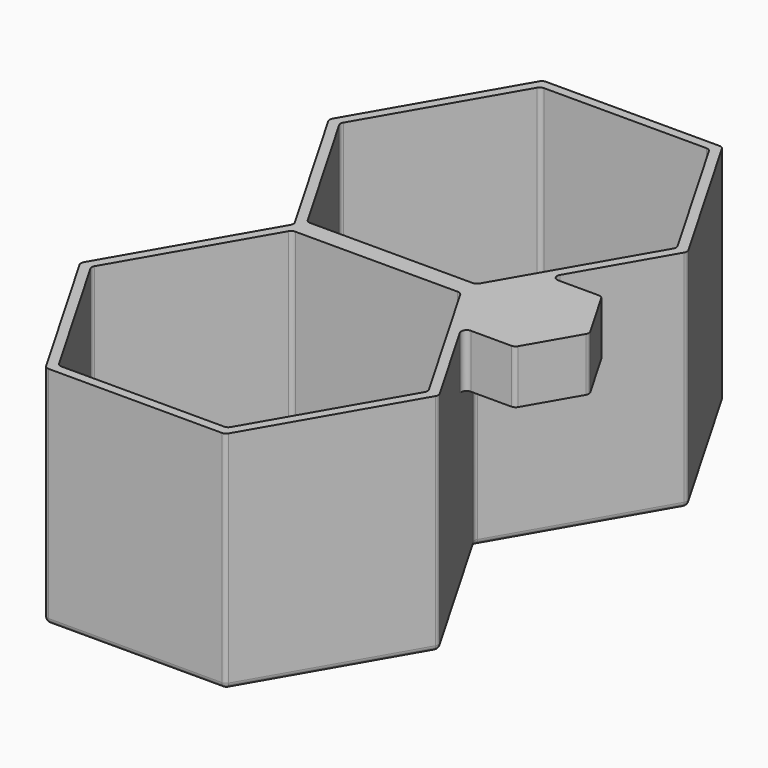
from build123d import *

# Parameters (mm, degrees)
F1_DEPTH = 42
F3_DEPTH = 40
F5_DEPTH = 10
F6_T     = -1.5
F7_R     = 1


# Not quite as in the source:
# - a shell that OpenCascade refuses in one call is made with other operations: the cavity is built on its own and cut out


with BuildPart() as f1:
    # F0 (on Top) → F1 (new body)
    with BuildSketch(Plane.XY):
        Polygon((-33.486315613, 29), (-16.7431578065, 0), (-33.486315613, -29), (-16.7431578065, -58), (16.7431578065, -58), (33.486315613, -29), (16.7431578065, 0), (33.486315613, 29), (16.7431578065, 58), (-16.7431578065, 58), align=None)
    extrude(amount=F1_DEPTH)

    # F2 (on face) → F3 (cut)
    with BuildSketch(Plane.XY.offset(42)):
        Polygon((15.7327948354, -1.75), (0, -1.75), (-15.7327948354, -1.75), (-31.4655896708, -29), (-15.7327948354, -56.25), (15.7327948354, -56.25), (31.4655896708, -29), align=None)
        Polygon((-15.7327948354, 1.75), (0, 1.75), (15.7327948354, 1.75), (31.4655896708, 29), (15.7327948354, 56.25), (-15.7327948354, 56.25), (-31.4655896708, 29), align=None)
    extrude(amount=-F3_DEPTH, mode=Mode.SUBTRACT)

    # F4 (on face) → F5 (join)
    with BuildSketch(Plane.XY.offset(42)):
        Polygon((32.4877562844, 10.1850116625), (20.7271178342, 10.1850116625), (14.8467986091, 0), (20.7271178342, -10.1850116625), (32.4877562844, -10.1850116625), (38.3680755094, 0), align=None)
    extrude(amount=-F5_DEPTH)

    # F6: a shell. OpenCascade refuses it in one call, so the cavity is built on its own and cut out:
    # the body offset inwards by the wall thickness, plus a prism from it out through each open face.
    f6_core = offset(f1.part, amount=F6_T, kind=Kind.INTERSECTION, mode=Mode.PRIVATE)
    f6_exits = [f6_core.faces().sort_by_distance(p)[0] for p in [
        (26.515913, 0, 33.5),
    ]]
    add(f6_core, mode=Mode.SUBTRACT)
    extrude(f6_exits, amount=-F6_T, mode=Mode.SUBTRACT)

    # F7
    f7_edges = [f1.edges().sort_by_distance(p)[0] for p in [
        (-33.486316, -29, 21),
        (-16.743158, 0, 21),
        (-33.486316, 29, 21),
        (-16.743158, 58, 21),
        (-16.743158, -58, 21),
        (16.743158, -58, 21),
        (33.486316, -29, 21),
        (16.743158, 0, 16),
        (33.486316, 29, 21),
        (16.743158, 58, 21),
        (-31.46559, 29, 22),
        (-15.732795, 56.25, 22),
        (15.732795, 56.25, 22),
        (31.46559, 29, 22),
        (15.732795, 1.75, 22),
        (-15.732795, 1.75, 22),
        (-31.46559, -29, 22),
        (-15.732795, -1.75, 22),
        (15.732795, -1.75, 22),
        (31.46559, -29, 22),
        (15.732795, -56.25, 22),
        (-15.732795, -56.25, 22),
        (0, 1.75, 2),
        (23.599192, 15.375, 2),
        (23.599192, 42.625, 2),
        (0, 56.25, 2),
        (-23.599192, 42.625, 2),
        (-23.599192, 15.375, 2),
        (0, -1.75, 2),
        (-23.599192, -15.375, 2),
        (-23.599192, -42.625, 2),
        (0, -56.25, 2),
        (23.599192, -42.625, 2),
        (23.599192, -15.375, 2),
        (-25.114737, 14.5, 0),
        (-25.114737, -14.5, 0),
        (-25.114737, -43.5, 0),
        (0, -58, 0),
        (25.114737, -43.5, 0),
        (25.114737, -14.5, 0),
        (25.114737, 14.5, 0),
        (25.114737, 43.5, 0),
        (0, 58, 0),
        (-25.114737, 43.5, 0),
        (22.623477, 10.185012, 37),
        (32.487756, 10.185012, 37),
        (38.368076, 0, 37),
        (32.487756, -10.185012, 37),
        (22.623477, -10.185012, 37),
    ]]
    fillet(f7_edges, radius=F7_R)


solid = f1.part
